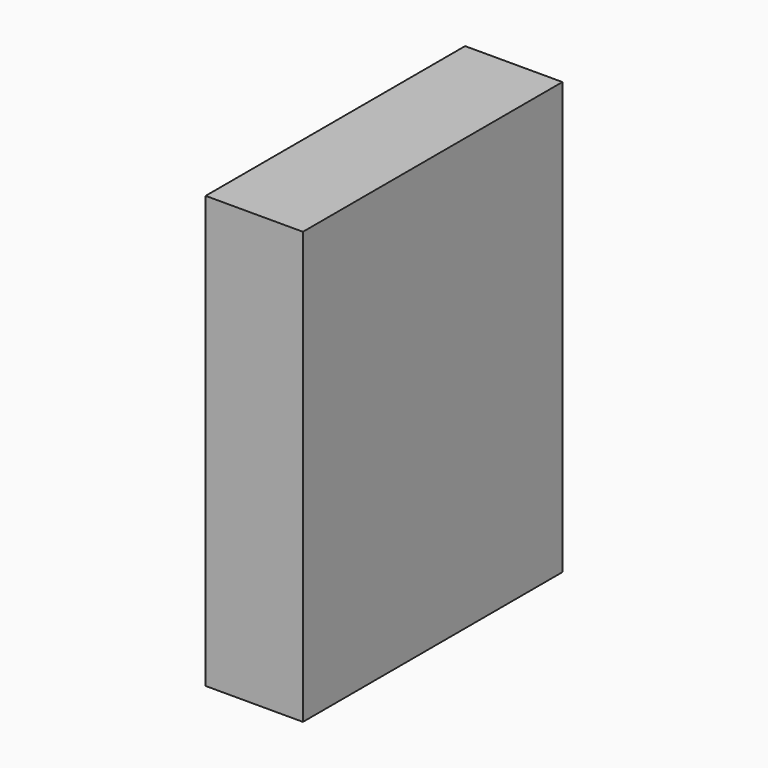
from build123d import *

# Parameters (mm, degrees)
F0_W     = 15.2400135994
F0_H     = 67.5844997168
F1_DEPTH = 50.8


# Not quite as in the source:
# - a feature names something its author has since deleted; it is built from what else it names


with BuildPart() as f1:
    # F0 (on Front) → F1 (new body)
    with BuildSketch(Plane.XZ):
        with Locations((7.6200067997, 55.8694899082)):
            Rectangle(F0_W, F0_H)
    extrude(amount=-F1_DEPTH)


solid = f1.part
